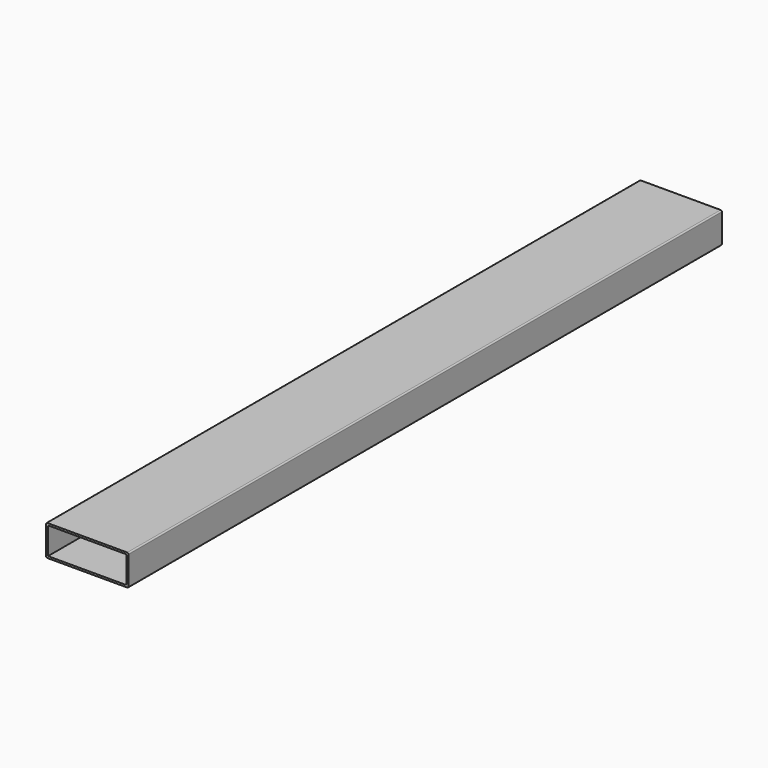
from build123d import *

# Parameters (mm, degrees)
F0_W     = 193.6623
F0_H     = 66.6623
F1_DEPTH = 914.4
F2_R     = 3.175


with BuildPart() as f1:
    # F0 (on Front) → F1 (new body, symmetric)
    with BuildSketch(Plane.XZ):
        Polygon((198.4248, -4.7752), (198.4248, 66.6623), (198.4248, 71.4248), (-4.7752, 71.4248), (-4.7752, -4.7752), align=None)
        with Locations((96.83115, 33.33115)):
            Rectangle(F0_W, F0_H, mode=Mode.SUBTRACT)
    extrude(amount=F1_DEPTH, both=True)

    # F2
    f2_edges = [f1.edges().sort_by_distance(p)[0] for p in [
        (-4.7752, 0, 71.4248),
        (0, 0, 66.6623),
        (-4.7752, 0, -4.7752),
        (198.4248, 0, -4.7752),
        (198.4248, 0, 71.4248),
        (193.6623, 0, 0),
        (193.6623, 0, 66.6623),
    ]]
    fillet(f2_edges, radius=F2_R)


solid = f1.part
